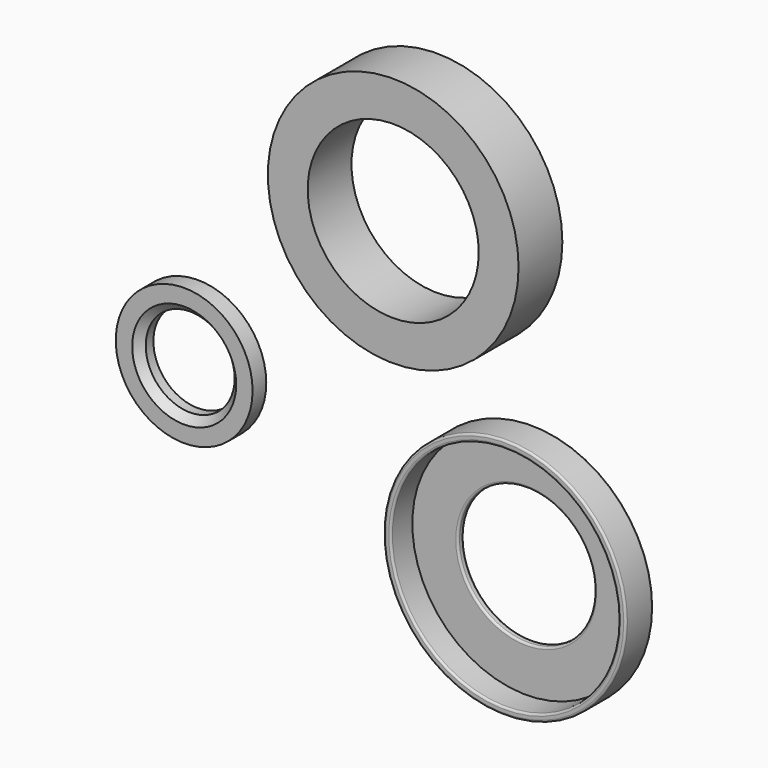
from build123d import *

# Parameters (mm, degrees)
F0_R            = 44.9834
F0_R_2          = 38.6334
F1_DEPTH        = 12.7
F2_T            = -2.70002
F3_R            = 25.4
F4_DEPTH        = 25.4
F5_R            = 0.762
F6_R            = 25.4
F6_R_2          = 16.51
F7_DEPTH        = 6.35
F8_SIZE         = 2.794
F9_R            = 46.5455
F9_R_2          = 31.75
F10_DEPTH       = 20.32
F11_W           = 44.5577651262
F11_H           = 45.586027205
F12_DEPTH       = 25.4
F14_D           = 25.4
F14_DEPTH       = 50.8
F14_CSINK_D     = 37.74948
F14_CSINK_ANGLE = 90
F14_TIP         = 7.6309298617


with BuildPart() as f1:
    # F0 (on Front) → F1 (new body)
    with BuildSketch(Plane.XZ):
        Circle(F0_R)
        Circle(F0_R_2, mode=Mode.SUBTRACT)
        Circle(F0_R_2)
    extrude(amount=F1_DEPTH)

    # F2
    f2_openings = [f1.faces().sort_by_distance(p)[0] for p in [
        (0, -12.7, 0),
    ]]
    offset(amount=F2_T, openings=f2_openings)

    # F3 (on face) → F4 (cut)
    with BuildSketch(Plane(origin=(0, 0, 0), x_dir=(-1, 0, 0), z_dir=(0, 1, 0))):
        Circle(F3_R)
    extrude(amount=-F4_DEPTH, mode=Mode.SUBTRACT)

    # F5
    f5_edges = [f1.edges().sort_by_distance(p)[0] for p in [
        (-44.9834, -12.7, 0),
        (-42.28338, -12.7, 0),
        (-44.9834, 0, 0),
        (25.4, 0, 0),
        (25.4, -2.70002, 0),
    ]]
    fillet(f5_edges, radius=F5_R)


with BuildPart() as f7:
    # F6 (on Front) → F7 (new body)
    with BuildSketch(Plane.XZ):
        with Locations((-124.0749135613, 26.5214759856)):
            Circle(F6_R)
        with Locations((-124.0749135613, 26.5214759856)):
            Circle(F6_R_2, mode=Mode.SUBTRACT)
    extrude(amount=F7_DEPTH)

    # F8
    f8_edges = [f7.edges().sort_by_distance(p)[0] for p in [
        (-140.584914, -6.35, 26.521476),
    ]]
    chamfer(f8_edges, length=F8_SIZE)


with BuildPart() as f10:
    # F9 (on Front) → F10 (new body)
    with BuildSketch(Plane.XZ):
        with Locations((-35.2853350341, 108.3141416311)):
            Circle(F9_R)
        with Locations((-35.2853350341, 108.3141416311)):
            Circle(F9_R_2, mode=Mode.SUBTRACT)
    extrude(amount=F10_DEPTH)


with BuildPart() as f12:
    # F11 (on Front) → F12 (new body)
    with BuildSketch(Plane.XZ):
        with Locations((135.7298120856, 15.5952200294)):
            Rectangle(F11_W, F11_H)
    extrude(amount=F12_DEPTH)

    # F14
    with Locations(Plane.XZ.offset(25.4)):
        with Locations((135.7298120856, 15.5952200294)):
            CounterSinkHole(F14_D / 2, F14_CSINK_D / 2, depth=F14_DEPTH, counter_sink_angle=F14_CSINK_ANGLE)
            with Locations((0, 0, -(F14_DEPTH + F14_TIP / 2))):  # 118° drill point
                Cone(0, F14_D / 2, F14_TIP, mode=Mode.SUBTRACT)


solid = Compound([f1.part, f7.part, f10.part])
